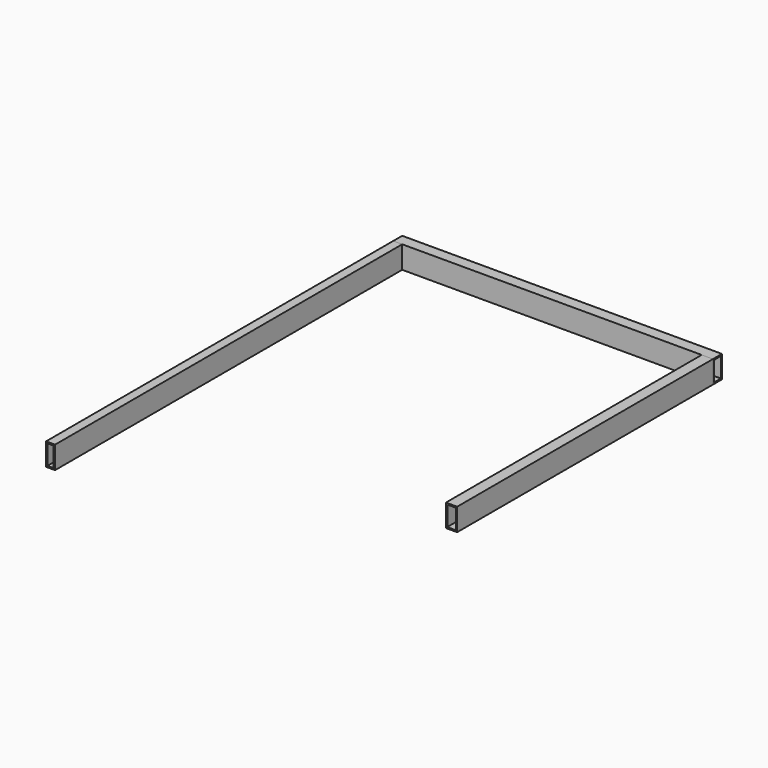
from build123d import *

# Parameters (mm, degrees)
F0_W     = 20
F0_H     = 50
F0_W_2   = 14
F0_H_2   = 44
F1_DEPTH = 965.2
F5_W     = 25
F5_H     = 50
F5_W_2   = 19
F5_H_2   = 44
F6_DEPTH = 711.2
F7_W     = 25
F7_H     = 50
F7_W_2   = 19
F7_H_2   = 44
F8_DEPTH = 711.2


# Not quite as in the source:
# - a feature of the source that left no trace in its solid (it failed there, or was rolled back) is left out


with BuildPart() as f1:
    # F0 (on Front) → F1 (new body)
    with BuildSketch(Plane.XZ):
        with Locations((-10, 25)):
            Rectangle(F0_W, F0_H)
        with Locations((-10, 25)):
            Rectangle(F0_W_2, F0_H_2, mode=Mode.SUBTRACT)
    extrude(amount=F1_DEPTH)


with BuildPart() as f2_1:
    # F2: copy of F1
    add(f1.part)


with BuildPart() as f6:
    # F5 (on face) → F6 (new body)
    with BuildSketch(Plane(origin=(-20, 0, 0), x_dir=(0, -1, 0), z_dir=(-1, 0, 0))):
        with Locations((-12.5, 25)):
            Rectangle(F5_W, F5_H)
        with Locations((-12.5, 25)):
            Rectangle(F5_W_2, F5_H_2, mode=Mode.SUBTRACT)
    extrude(amount=-F6_DEPTH)


with BuildPart() as f8:
    # F7 (on face) → F8 (new body)
    with BuildSketch(Plane.XZ):
        with Locations((678.7, 25)):
            Rectangle(F7_W, F7_H)
        with Locations((678.7, 25)):
            Rectangle(F7_W_2, F7_H_2, mode=Mode.SUBTRACT)
    extrude(amount=F8_DEPTH)


solid = Compound([f1.part, f2_1.part, f6.part, f8.part])
